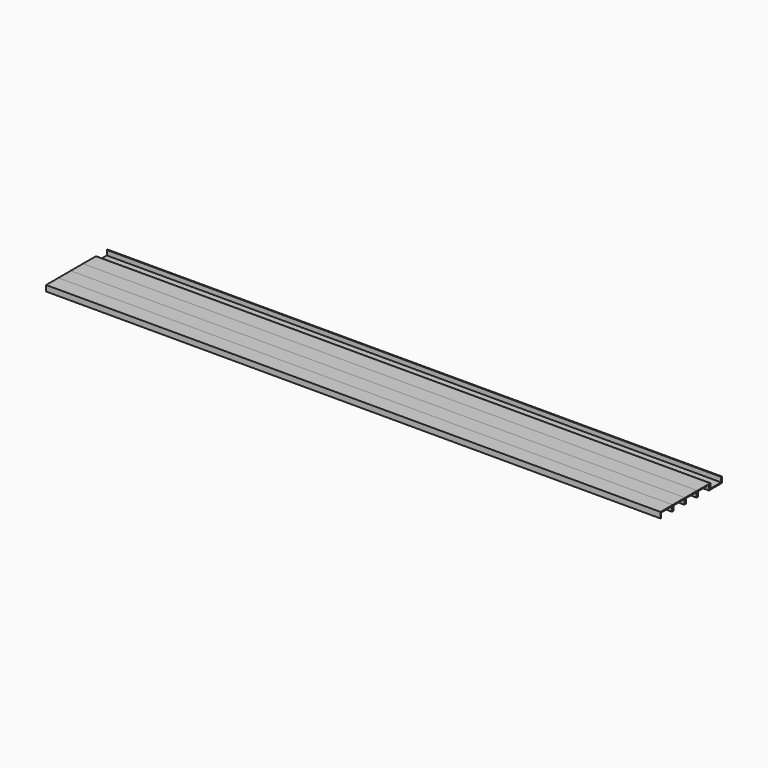
from build123d import *

# Parameters (mm, degrees)
F1_DEPTH = 8000
F2_DEPTH = 8000
F3_DEPTH = 8000
F4_DEPTH = 8000
F5_DEPTH = 8000


# Not quite as in the source:
# - a feature of the source that left no trace in its solid (it failed there, or was rolled back) is left out


with BuildPart() as f1:
    # F0 (on Right) → F1 (new body)
    with BuildSketch(Plane.YZ):
        Polygon((0, -75), (0, 0), (-12, 0), (-12, -63), (-188, -63), (-188, 0), (-200, 0), (-200, -75), align=None)
    extrude(amount=F1_DEPTH)


with BuildPart() as f2:
    # F0 (on Right) → F2 (new body)
    with BuildSketch(Plane.YZ):
        Polygon((-212, -75), (-200, -75), (-200, 0), (-400, 0), (-400, -75), (-388, -75), (-388, -12), (-212, -12), align=None)
    extrude(amount=F2_DEPTH)


with BuildPart() as f3:
    # F0 (on Right) → F3 (new body)
    with BuildSketch(Plane.YZ):
        Polygon((-400, -75), (-400, 0), (-600, 0), (-600, -75), (-588, -75), (-588, -12), (-412, -12), (-412, -75), align=None)
    extrude(amount=F3_DEPTH)


with BuildPart() as f4:
    # F0 (on Right) → F4 (new body)
    with BuildSketch(Plane.YZ):
        Polygon((-600, -75), (-600, 0), (-800, 0), (-800, -75), (-788, -75), (-788, -12), (-612, -12), (-612, -75), align=None)
    extrude(amount=F4_DEPTH)


with BuildPart() as f5:
    # F0 (on Right) → F5 (new body)
    with BuildSketch(Plane.YZ):
        Polygon((-800, -75), (-800, 0), (-812, 0), (-988, 0), (-1000, 0), (-1000, -75), (-988, -75), (-988, -12), (-812, -12), (-812, -75), align=None)
    extrude(amount=F5_DEPTH)


solid = Compound([f1.part, f2.part, f3.part, f4.part, f5.part])
